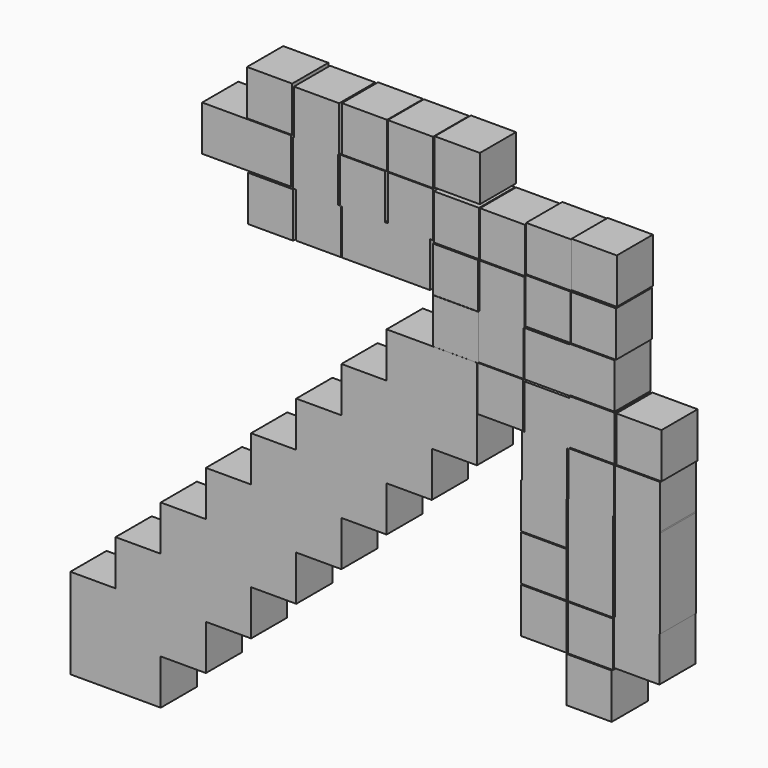
from build123d import *

# Parameters (mm, degrees)
F0_W     = 12.7
F0_H     = 12.7
F1_DEPTH = 12.7
F0_W_2   = 0.2243827701
F0_H_2   = 0.051115793
F0_W_3   = 12.4972398996
F0_H_3   = 0.1287359416
F0_W_4   = 0.3314997673
F0_H_4   = 0.1984063208
F0_W_5   = 11.8897642612
F0_H_5   = 0.1287396669
F0_W_6   = 0.1287322164
F0_H_6   = 12.2248056948
F0_H_7   = 0.534263593
F0_H_8   = 0.1287364073
F0_H_9   = 12.5712635927
F0_H_10  = 12.4972361743
F0_H_11  = 0.128736873
F0_W_7   = 12.4972324491
F0_H_12  = 0.1287373386
F0_W_8   = 11.8397336125
F0_H_13  = 0.0830378056
F0_W_9   = 12.0437275618
F0_H_14  = 12.6169621944
F0_W_10  = 0.0827565461
F0_W_11  = 0.3695247367
F0_W_12  = 11.8397359408
F0_W_13  = 12.4132522985
F0_H_15  = 0.083030355
F0_W_14  = 0.3695140265
F0_W_15  = 12.3304859735


# Not quite as in the source:
# - ends of sketch curves that miss each other by under 0.0002 mm in the source are joined


with BuildPart() as f1:
    # F0 (on Front) → F1 (new body)
    with BuildSketch(Plane.XZ):
        with Locations((19.4921738029, 7.627361536)):
            Rectangle(F0_W, F0_H)
        with Locations((6.7921738029, -5.072638464)):
            Rectangle(F0_W, F0_H)
        with Locations((6.7921738029, 7.627361536)):
            Rectangle(F0_W, F0_H)
        with Locations((19.4921738029, 20.327361536)):
            Rectangle(F0_W, F0_H)
        with Locations((32.1921738029, 20.327361536)):
            Rectangle(F0_W, F0_H)
        with Locations((-5.9078261971, 7.627361536)):
            Rectangle(F0_W, F0_H)
        with Locations((-5.9078261971, -5.072638464)):
            Rectangle(F0_W, F0_H)
        with Locations((6.7921738029, 20.327361536)):
            Rectangle(F0_W, F0_H)
        with Locations((32.1921738029, 33.027361536)):
            Rectangle(F0_W, F0_H)
        with Locations((19.4921738029, 33.027361536)):
            Rectangle(F0_W, F0_H)
        with Locations((-18.6078261971, -5.072638464)):
            Rectangle(F0_W, F0_H)
        with Locations((-5.9078261971, -17.772638464)):
            Rectangle(F0_W, F0_H)
        Polygon((38.5421738029, 39.377361536), (38.5421738029, 26.677361536), (51.2421738029, 26.677361536), (51.2421738029, 52.077361536), (25.8421738029, 52.077361536), (25.8421738029, 39.377361536), align=None)
        with Locations((-18.6078261971, -17.772638464)):
            Rectangle(F0_W, F0_H)
        with Locations((-31.3078261971, -17.772638464)):
            Rectangle(F0_W, F0_H)
        with Locations((-18.6078261971, -30.472638464)):
            Rectangle(F0_W, F0_H)
        with Locations((-31.3078261971, -30.472638464)):
            Rectangle(F0_W, F0_H)
        with Locations((-44.0078261971, -30.472638464)):
            Rectangle(F0_W, F0_H)
        with Locations((-31.3078261971, -43.172638464)):
            Rectangle(F0_W, F0_H)
        with Locations((-44.0078261971, -43.172638464)):
            Rectangle(F0_W, F0_H)
        Polygon((-50.3578261971, -49.522638464), (-50.3578261971, -36.822638464), (-63.0578261971, -36.822638464), (-63.0578261971, -62.222638464), (-37.6578261971, -62.222638464), (-37.6578261971, -49.522638464), align=None)
    extrude(amount=F1_DEPTH)


with BuildPart() as f1b:
    # F0 (on Front) → F1, piece 2 (new body)
    with BuildSketch(Plane.XZ):
        Polygon((51.6497982502, 52.1384445786), (51.6497982502, 52.0873287857), (51.4254154801, 52.0873287857), (51.4254154801, 39.4384445786), (64.1254154801, 39.4384445786), (64.1254154801, 52.1384445786), align=None)
        with Locations((51.5376068652, 52.1128866822)):
            Rectangle(F0_W_2, F0_H_2)
        Polygon((38.9497982502, 52.0873287857), (51.4254154801, 52.0873287857), (51.4254154801, 52.1384445786), (51.6497982502, 52.1384445786), (51.6497982502, 64.7873287857), (38.9497982502, 64.7873287857), align=None)
    extrude(amount=F1_DEPTH)


with BuildPart() as f1c:
    # F0 (on Front) → F1, piece 3 (new body)
    with BuildSketch(Plane.XZ):
        with Locations((45.2457629144, 71.2007209659)):
            Rectangle(F0_W, F0_H)
    extrude(amount=F1_DEPTH)


with BuildPart() as f1d:
    # F0 (on Front) → F1, piece 4 (new body)
    with BuildSketch(Plane.XZ):
        Polygon((51.6984755337, 52.3428389966), (64.3984755337, 52.3428389966), (64.3984755337, 64.914103055), (51.9012356341, 64.914103055), (51.9012356341, 65.0428389966), (51.6984755337, 65.0428389966), align=None)
        with Locations((58.1498555839, 64.9784710258)):
            Rectangle(F0_W_3, F0_H_3)
        Polygon((64.3984755337, 65.0428389966), (64.3984755337, 64.914103055), (64.6012356341, 64.914103055), (64.6012356341, 77.614103055), (51.9012356341, 77.614103055), (51.9012356341, 65.0428389966), align=None)
    extrude(amount=F1_DEPTH)


with BuildPart() as f1e:
    # F0 (on Front) → F1, piece 5 (new body)
    with BuildSketch(Plane.XZ):
        Polygon((77.3752597928, 39.2920268536), (77.3752597928, 39.0936205328), (77.0437600255, 39.0936205328), (77.0437600255, 26.7207665205), (89.5409999251, 26.7207665205), (89.5409999251, 26.5920268536), (89.7437600255, 26.5920268536), (89.7437600255, 39.2920268536), align=None)
        with Locations((77.2095099092, 39.1928236932)):
            Rectangle(F0_W_4, F0_H_4)
        Polygon((76.5650240541, 39.0936205328), (77.0437600255, 39.0936205328), (77.0437600255, 39.2920268536), (77.3752597928, 39.2920268536), (77.3752597928, 39.5688148379), (77.2465275764, 39.5688148379), (77.2465275764, 51.7936205328), (64.6752597928, 51.7936205328), (64.6752597928, 39.2920268536), (76.5650240541, 39.2920268536), align=None)
        Polygon((76.5650240541, 26.5920268536), (76.5650240541, 39.0936205328), (64.6752597928, 39.0936205328), (64.6752597928, 39.2920268536), (63.8650240541, 39.2920268536), (63.8650240541, 27.1262904465), (76.3622639537, 27.1262904465), (76.3622639537, 26.5920268536), align=None)
        with Locations((70.6201419234, 39.1928236932)):
            Rectangle(F0_W_5, F0_H_4)
        with Locations((83.2923799753, 26.656396687)):
            Rectangle(F0_W_3, F0_H_5)
        Polygon((77.0437600255, 26.5920268536), (77.0437600255, 26.7207665205), (76.8409999251, 26.7207665205), (76.8409999251, 14.1495029278), (89.5409999251, 14.1495029278), (89.5409999251, 26.5920268536), align=None)
        with Locations((77.3108936846, 45.6812176853)):
            Rectangle(F0_W_6, F0_H_6)
        Polygon((77.3752597928, 51.7936205328), (77.3752597928, 39.5688148379), (89.9465275764, 39.5688148379), (89.9465275764, 52.2688148379), (77.2465275764, 52.2688148379), (77.2465275764, 51.7936205328), align=None)
        with Locations((70.1136440039, 26.85915865)):
            Rectangle(F0_W_3, F0_H_7)
        Polygon((76.3622639537, 14.4262904465), (76.3622639537, 26.5920268536), (63.8650240541, 26.5920268536), (63.8650240541, 27.1262904465), (63.6622639537, 27.1262904465), (63.6622639537, 14.4262904465), align=None)
        with Locations((83.1909999251, 14.0851347242)):
            Rectangle(F0_W, F0_H_8)
        with Locations((83.1909999251, 7.7351347242)):
            Rectangle(F0_W, F0_H_9)
    extrude(amount=F1_DEPTH)


with BuildPart() as f1f:
    # F0 (on Front) → F1, piece 6 (new body)
    with BuildSketch(Plane.XZ):
        Polygon((64.6752597928, 52.3428389966), (77.3752597928, 52.3428389966), (77.3752597928, 52.5456028223), (77.2465275764, 52.5456028223), (77.2465275764, 65.0428389966), (64.6752597928, 65.0428389966), align=None)
        with Locations((77.3108936846, 58.7942209095)):
            Rectangle(F0_W_6, F0_H_10)
        Polygon((77.3752597928, 65.0428389966), (77.3752597928, 52.5456028223), (89.9465275764, 52.5456028223), (89.9465275764, 65.2456028223), (77.2465275764, 65.2456028223), (77.2465275764, 65.0428389966), align=None)
    extrude(amount=F1_DEPTH)


with BuildPart() as f1g:
    # F0 (on Front) → F1, piece 7 (new body)
    with BuildSketch(Plane.XZ):
        with Locations((71.2280273438, 71.8723908067)):
            Rectangle(F0_W, F0_H)
    extrude(amount=F1_DEPTH)


with BuildPart() as f1h:
    # F0 (on Front) → F1, piece 8 (new body)
    with BuildSketch(Plane.XZ):
        with Locations((84.0020477772, 71.8723908067)):
            Rectangle(F0_W, F0_H)
    extrude(amount=F1_DEPTH)


with BuildPart() as f1i:
    # F0 (on Front) → F1, piece 9 (new body)
    with BuildSketch(Plane.XZ):
        with Locations((84.2048153281, 85.0519388914)):
            Rectangle(F0_W, F0_H)
    extrude(amount=F1_DEPTH)


with BuildPart() as f1j:
    # F0 (on Front) → F1, piece 10 (new body)
    with BuildSketch(Plane.XZ):
        with Locations((83.1909999251, -5.1772845909)):
            Rectangle(F0_W, F0_H)
    extrude(amount=F1_DEPTH)


with BuildPart() as f1k:
    # F0 (on Front) → F1, piece 11 (new body)
    with BuildSketch(Plane.XZ):
        with Locations((71.4307874441, 84.849178791)):
            Rectangle(F0_W, F0_H)
    extrude(amount=F1_DEPTH)


with BuildPart() as f1l:
    # F0 (on Front) → F1, piece 12 (new body)
    with BuildSketch(Plane.XZ):
        with Locations((58.4539994597, 84.2408910394)):
            Rectangle(F0_W, F0_H)
    extrude(amount=F1_DEPTH)


with BuildPart() as f1m:
    # F0 (on Front) → F1, piece 13 (new body)
    with BuildSketch(Plane.XZ):
        Polygon((102.7219263673, 1.6522653565), (102.7219263673, 14.2235284835), (90.0219263673, 14.2235284835), (90.0219263673, 1.7810026951), (102.5191588163, 1.7810026951), (102.5191588163, 1.6522653565), align=None)
        with Locations((96.3719263673, 14.28789692)):
            Rectangle(F0_W, F0_H_11)
        Polygon((90.0219263673, 14.3522653565), (102.7219263673, 14.3522653565), (102.7219263673, 26.5920268536), (90.0219189167, 26.5920268536), align=None)
        Polygon((90.0219263673, 1.6522653565), (90.0219263673, 1.7810026951), (89.8191588163, 1.7810026951), (89.8191588163, -10.9189973049), (102.5191588163, -10.9189973049), (102.5191588163, 1.6522653565), align=None)
        with Locations((96.2705425918, 1.7166340258)):
            Rectangle(F0_W_7, F0_H_12)
        Polygon((90.0219189167, 26.5920268536), (102.7219189167, 26.5920268536), (102.7219263673, 26.9235284835), (90.0219263673, 26.9235284835), align=None)
        Polygon((90.0219263673, 26.9235284835), (102.7219263673, 26.9235284835), (102.7219189167, 39.2920268536), (90.0219189167, 39.2920268536), align=None)
    extrude(amount=F1_DEPTH)


with BuildPart() as f1n:
    # F0 (on Front) → F1, piece 14 (new body)
    with BuildSketch(Plane.XZ):
        with Locations((82.7854722738, -18.1540716439)):
            Rectangle(F0_W, F0_H)
    extrude(amount=F1_DEPTH)


with BuildPart() as f1o:
    # F0 (on Front) → F1, piece 15 (new body)
    with BuildSketch(Plane.XZ):
        with Locations((70.0122639537, -5.1772845909)):
            Rectangle(F0_W, F0_H)
    extrude(amount=F1_DEPTH)


with BuildPart() as f1p:
    # F0 (on Front) → F1, piece 16 (new body)
    with BuildSketch(Plane.XZ):
        with Locations((70.0122639537, 7.7995029278)):
            Rectangle(F0_W, F0_H)
    extrude(amount=F1_DEPTH)


with BuildPart() as f1q:
    # F0 (on Front) → F1, piece 17 (new body)
    with BuildSketch(Plane.XZ):
        Polygon((38.0208572209, 78.3694865346), (38.8811236084, 78.3694865346), (38.8811236084, 91.0694865346), (26.1811236084, 91.0694865346), (26.1811236084, 78.4525243402), (38.0208572209, 78.4525243402), align=None)
        Polygon((38.0208572209, 65.7525243402), (38.0208572209, 78.3694865346), (26.1811236084, 78.3694865346), (26.1811236084, 78.4525243402), (25.9771296591, 78.4525243402), (25.9771296591, 65.7525243402), align=None)
        with Locations((32.1009904146, 78.4110054374)):
            Rectangle(F0_W_8, F0_H_13)
        Polygon((25.3208572209, 65.7525243402), (25.9771296591, 65.7525243402), (25.9771296591, 78.4525243402), (25.403613767, 78.4525243402), (25.403613767, 78.3694865346), (25.3208572209, 78.3694865346), align=None)
        with Locations((19.29899344, 72.0610054374)):
            Rectangle(F0_W_9, F0_H_14)
        Polygon((25.3208572209, 78.4525243402), (25.403613767, 78.4525243402), (25.403613767, 91.0694865346), (12.703613767, 91.0694865346), (12.703613767, 78.4525243402), (13.0731385037, 78.4525243402), (13.0731385037, 78.3694865346), (13.2771296591, 78.3694865346), (13.2771296591, 78.4525243402), align=None)
        with Locations((25.362235494, 78.4110054374)):
            Rectangle(F0_W_10, F0_H_13)
        with Locations((19.29899344, 78.4110054374)):
            Rectangle(F0_W_9, F0_H_13)
        Polygon((13.0731385037, 65.7525243402), (13.0731385037, 78.3694865346), (12.703613767, 78.3694865346), (12.703613767, 78.4525243402), (12.2128744446, 78.4525243402), (12.2128744446, 78.3694865346), (0.3731385037, 78.3694865346), (0.3731385037, 65.7525243402), align=None)
        with Locations((12.8883761354, 78.4110054374)):
            Rectangle(F0_W_11, F0_H_13)
        Polygon((0.3731385037, 78.4525243402), (12.2128744446, 78.4525243402), (12.2128744446, 90.9864561796), (-0.200377854, 90.9864561796), (-0.200377854, 91.0694865346), (-0.4871255554, 91.0694865346), (-0.4871255554, 78.3694865346), (0.3731385037, 78.3694865346), align=None)
        with Locations((6.2930064742, 78.4110054374)):
            Rectangle(F0_W_12, F0_H_13)
        with Locations((6.0062482953, 91.0279713571)):
            Rectangle(F0_W_13, F0_H_15)
        Polygon((12.2128744446, 91.0694865346), (12.2128744446, 90.9864561796), (12.499622146, 90.9864561796), (12.499622146, 103.6864561796), (-0.200377854, 103.6864561796), (-0.200377854, 91.0694865346), align=None)
    extrude(amount=F1_DEPTH)


with BuildPart() as f1r:
    # F0 (on Front) → F1, piece 18 (new body)
    with BuildSketch(Plane.XZ):
        with Locations((45.4774945974, 84.2408910394)):
            Rectangle(F0_W, F0_H)
    extrude(amount=F1_DEPTH)


with BuildPart() as f1s:
    # F0 (on Front) → F1, piece 19 (new body)
    with BuildSketch(Plane.XZ):
        with Locations((-13.4931176435, 85.0062444806)):
            Rectangle(F0_W_14, F0_H)
        with Locations((-7.1431176435, 85.0062444806)):
            Rectangle(F0_W_15, F0_H)
        with Locations((-19.8431176435, 85.0062444806)):
            Rectangle(F0_W_15, F0_H)
    extrude(amount=F1_DEPTH)


with BuildPart() as f1t:
    # F0 (on Front) → F1, piece 20 (new body)
    with BuildSketch(Plane.XZ):
        with Locations((-6.7543690093, 71.8157812953)):
            Rectangle(F0_W, F0_H)
    extrude(amount=F1_DEPTH)


with BuildPart() as f1u:
    # F0 (on Front) → F1, piece 21 (new body)
    with BuildSketch(Plane.XZ):
        with Locations((96.7774540186, 45.9188148379)):
            Rectangle(F0_W, F0_H)
    extrude(amount=F1_DEPTH)


with BuildPart() as f1v:
    # F0 (on Front) → F1, piece 22 (new body)
    with BuildSketch(Plane.XZ):
        with Locations((19.6271296591, 97.6231992245)):
            Rectangle(F0_W, F0_H)
    extrude(amount=F1_DEPTH)


with BuildPart() as f1w:
    # F0 (on Front) → F1, piece 23 (new body)
    with BuildSketch(Plane.XZ):
        with Locations((-7.0411167108, 97.9099571705)):
            Rectangle(F0_W, F0_H)
    extrude(amount=F1_DEPTH)


with BuildPart() as f1x:
    # F0 (on Front) → F1, piece 24 (new body)
    with BuildSketch(Plane.XZ):
        with Locations((45.7218587399, 97.9099571705)):
            Rectangle(F0_W, F0_H)
    extrude(amount=F1_DEPTH)


with BuildPart() as f1y:
    # F0 (on Front) → F1, piece 25 (new body)
    with BuildSketch(Plane.XZ):
        with Locations((32.5311236084, 97.6231992245)):
            Rectangle(F0_W, F0_H)
    extrude(amount=F1_DEPTH)


solid = Compound([f1.part, f1b.part, f1c.part, f1d.part, f1e.part, f1f.part, f1g.part, f1h.part, f1i.part, f1j.part, f1k.part, f1l.part, f1m.part, f1n.part, f1o.part, f1p.part, f1q.part, f1r.part, f1s.part, f1t.part, f1u.part, f1v.part, f1w.part, f1x.part, f1y.part])
